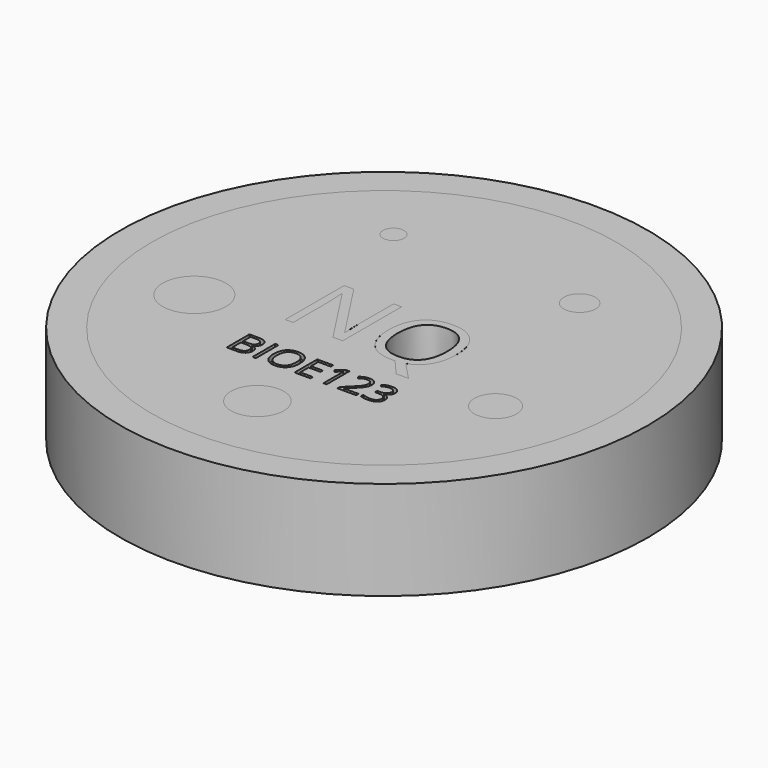
from build123d import *

# Parameters (mm, degrees)
F0_R         = 25
F1_DEPTH     = 3
F2_R         = 25
F2_R_2       = 22
F2_TEXT_SIZE = 9.7620500305
F3_DEPTH     = 6.35
F4_DEPTH     = 6.35
F5_TEXT_SIZE = 3.7660350712
F6_DEPTH     = 0.5


# Not quite as in the source:
# - Text() gives the source's letters only with a copy of the font that has no kerning and outlines rounded to 1/6400 em; it was checked with that copy


with BuildPart() as f1:
    # F0 (on Top) → F1 (new body)
    with BuildSketch(Plane.XY):
        Circle(F0_R)
    extrude(amount=F1_DEPTH)

    # F2 (on face) → F3 (join)
    with BuildSketch(Plane.XY.offset(3)):
        Circle(F2_R)
        Circle(F2_R_2, mode=Mode.SUBTRACT)
        with BuildLine():
            ThreePointArc((-9.6057533582, 11.5208290683), (-8.8167787844, 12.1352549156), (-7.9886185271, 12.6957462967))
            ThreePointArc((-7.9886185271, 12.6957462967), (-9.4045640367, 12.94427191), (-9.6057533582, 11.5208290683))
        make_face()
        with BuildLine():
            ThreePointArc((-9.6057533582, 11.5208290683), (-8.4919515794, 11.1894815353), (-7.8167787844, 12.1352549156))
            ThreePointArc((-7.8167787844, 12.1352549156), (-7.8607034063, 12.4283758315), (-7.9886185271, 12.6957462967))
            ThreePointArc((-7.9886185271, 12.6957462967), (-8.8167787844, 12.1352549156), (-9.6057533582, 11.5208290683))
        make_face()
        with BuildLine():
            ThreePointArc((9.9847025259, 11.1940035496), (8.8167787844, 12.1352549156), (7.560687255, 12.9551537325))
            ThreePointArc((7.560687255, 12.9551537325), (7.9351009059, 10.9217294241), (9.9847025259, 11.1940035496))
        make_face()
        with BuildLine():
            ThreePointArc((10.3167787844, 12.1352549156), (9.2444835342, 13.5729852961), (7.560687255, 12.9551537325))
            ThreePointArc((7.560687255, 12.9551537325), (8.8167787844, 12.1352549156), (9.9847025259, 11.1940035496))
            ThreePointArc((9.9847025259, 11.1940035496), (10.2313256398, 11.6361986123), (10.3167787844, 12.1352549156))
        make_face()
        with BuildLine():
            ThreePointArc((13.5223811584, -6.4919340574), (14.2658477444, -4.6352549156), (14.7556992594, -2.696171242))
            ThreePointArc((14.7556992594, -2.696171242), (12.3637347118, -4.0172209269), (13.5223811584, -6.4919340574))
        make_face()
        with BuildLine():
            ThreePointArc((16.2658477444, -4.6352549156), (15.8437740782, -3.4063739267), (14.7556992594, -2.696171242))
            ThreePointArc((14.7556992594, -2.696171242), (14.2658477444, -4.6352549156), (13.5223811584, -6.4919340574))
            ThreePointArc((13.5223811584, -6.4919340574), (15.3867997568, -6.2915962409), (16.2658477444, -4.6352549156))
        make_face()
        with BuildLine():
            ThreePointArc((2.4913043215, -14.7916666667), (0, -12.5), (-2.4913043215, -14.7916666667))
            ThreePointArc((-2.4913043215, -14.7916666667), (0, -15), (2.4913043215, -14.7916666667))
        make_face()
        with BuildLine():
            ThreePointArc((2.4913043215, -14.7916666667), (0, -15), (-2.4913043215, -14.7916666667))
            ThreePointArc((-2.4913043215, -14.7916666667), (-0.104257365, -17.4978251344), (2.5, -15))
            ThreePointArc((2.5, -15), (2.4978251344, -14.895742635), (2.4913043215, -14.7916666667))
        make_face()
        with BuildLine():
            ThreePointArc((-13.0581267078, -7.3814176744), (-14.2658477444, -4.6352549156), (-14.9029348713, -1.7036819602))
            ThreePointArc((-14.9029348713, -1.7036819602), (-17.1190172933, -5.5623058987), (-13.0581267078, -7.3814176744))
        make_face()
        with BuildLine():
            ThreePointArc((-11.2658477444, -4.6352549156), (-12.3831981993, -2.2995257596), (-14.9029348713, -1.7036819602))
            ThreePointArc((-14.9029348713, -1.7036819602), (-14.2658477444, -4.6352549156), (-13.0581267078, -7.3814176744))
            ThreePointArc((-13.0581267078, -7.3814176744), (-11.7535616232, -6.2748946459), (-11.2658477444, -4.6352549156))
        make_face()
        with Locations((-7.5, -3.5248006052)):
            Text('NQ', F2_TEXT_SIZE, font='Open Sans', text_align=(TextAlign.LEFT, TextAlign.BOTTOM))
    extrude(amount=F3_DEPTH)


with BuildPart() as f4:
    # F2 (on face) → F4 (new body)
    with BuildSketch(Plane.XY.offset(3)):
        Circle(F2_R_2)
        with BuildLine():
            ThreePointArc((-9.6057533582, 11.5208290683), (-9.4045640367, 12.94427191), (-7.9886185271, 12.6957462967))
            ThreePointArc((-7.9886185271, 12.6957462967), (-0.2502086086, 14.9979130432), (7.560687255, 12.9551537325))
            ThreePointArc((7.560687255, 12.9551537325), (9.2444835342, 13.5729852961), (10.3167787844, 12.1352549156))
            ThreePointArc((10.3167787844, 12.1352549156), (10.2313256398, 11.6361986123), (9.9847025259, 11.1940035496))
            ThreePointArc((9.9847025259, 11.1940035496), (13.6888739107, 6.1330849542), (15, 0))
            ThreePointArc((15, 0), (14.9387999667, -1.3536083461), (14.7556992594, -2.696171242))
            ThreePointArc((14.7556992594, -2.696171242), (15.8437740782, -3.4063739267), (16.2658477444, -4.6352549156))
            ThreePointArc((16.2658477444, -4.6352549156), (15.3867997568, -6.2915962409), (13.5223811584, -6.4919340574))
            ThreePointArc((13.5223811584, -6.4919340574), (9.0183657615, -11.9862036939), (2.4913043215, -14.7916666667))
            ThreePointArc((2.4913043215, -14.7916666667), (2.4978251344, -14.895742635), (2.5, -15))
            ThreePointArc((2.5, -15), (-0.104257365, -17.4978251344), (-2.4913043215, -14.7916666667))
            ThreePointArc((-2.4913043215, -14.7916666667), (-8.6124415159, -12.2811176664), (-13.0581267078, -7.3814176744))
            ThreePointArc((-13.0581267078, -7.3814176744), (-17.1190172933, -5.5623058987), (-14.9029348713, -1.7036819602))
            ThreePointArc((-14.9029348713, -1.7036819602), (-13.9244702832, 5.5775556771), (-9.6057533582, 11.5208290683))
        make_face(mode=Mode.SUBTRACT)
        with BuildLine():
            ThreePointArc((-7.9886185271, 12.6957462967), (-7.8607034063, 12.4283758315), (-7.8167787844, 12.1352549156))
            ThreePointArc((-7.8167787844, 12.1352549156), (-8.4919515794, 11.1894815353), (-9.6057533582, 11.5208290683))
            ThreePointArc((-9.6057533582, 11.5208290683), (-13.9244702832, 5.5775556771), (-14.9029348713, -1.7036819602))
            ThreePointArc((-14.9029348713, -1.7036819602), (-12.3831981993, -2.2995257596), (-11.2658477444, -4.6352549156))
            ThreePointArc((-11.2658477444, -4.6352549156), (-11.7535616232, -6.2748946459), (-13.0581267078, -7.3814176744))
            ThreePointArc((-13.0581267078, -7.3814176744), (-8.6124415159, -12.2811176664), (-2.4913043215, -14.7916666667))
            ThreePointArc((-2.4913043215, -14.7916666667), (0, -12.5), (2.4913043215, -14.7916666667))
            ThreePointArc((2.4913043215, -14.7916666667), (9.0183657615, -11.9862036939), (13.5223811584, -6.4919340574))
            ThreePointArc((13.5223811584, -6.4919340574), (12.3637347118, -4.0172209269), (14.7556992594, -2.696171242))
            ThreePointArc((14.7556992594, -2.696171242), (14.9387999667, -1.3536083461), (15, 0))
            ThreePointArc((15, 0), (13.6888739107, 6.1330849542), (9.9847025259, 11.1940035496))
            ThreePointArc((9.9847025259, 11.1940035496), (7.9351009059, 10.9217294241), (7.560687255, 12.9551537325))
            ThreePointArc((7.560687255, 12.9551537325), (-0.2502086086, 14.9979130432), (-7.9886185271, 12.6957462967))
        make_face()
        with BuildLine():
            Line((-1.0982306284, 3.4443879244), (-1.0982306284, -3.5248006052))
            Line((-1.0982306284, -3.5248006052), (-2.0225747407, -3.5248006052))
            Line((-2.0225747407, -3.5248006052), (-5.8312995729, 2.3232774912))
            Line((-5.8312995729, 2.3232774912), (-5.8694325808, 2.3232774912))
            add(Edge.make_bspline(
                [(-5.8694325808, 2.3232774912), (-5.793166565, 1.293686277), (-5.793166565, 0.4364562587)],
                knots=[0, 0, 0, 1, 1, 1], degree=2))
            Line((-5.793166565, 0.4364562587), (-5.793166565, -3.5248006052))
            Line((-5.793166565, -3.5248006052), (-6.5420988408, -3.5248006052))
            Line((-6.5420988408, -3.5248006052), (-6.5420988408, 3.4443879244))
            Line((-6.5420988408, 3.4443879244), (-5.6269066504, 3.4443879244))
            Line((-5.6269066504, 3.4443879244), (-1.8273337401, -2.3808103673))
            Line((-1.8273337401, -2.3808103673), (-1.7892007322, -2.3808103673))
            add(Edge.make_bspline(
                [(-1.7892007322, -2.3808103673), (-1.7983526541, -2.2526834606), (-1.831909701, -1.5540867553)],
                knots=[0, 0, 0, 1, 1, 1], degree=2))
            add(Edge.make_bspline(
                [(-1.831909701, -1.5540867553), (-1.865466748, -0.85549005), (-1.8563148261, -0.5550019475)],
                knots=[0, 0, 0, 1, 1, 1], degree=2))
            Line((-1.8563148261, -0.5550019475), (-1.8563148261, 3.4443879244))
            Line((-1.8563148261, 3.4443879244), (-1.0982306284, 3.4443879244))
        make_face(mode=Mode.SUBTRACT)
        with BuildLine():
            add(Edge.make_bspline(
                [(6.0234899329, 2.6008857889), (6.8669920683, 1.6475605907), (6.8669920683, -0.0302917583)],
                knots=[0, 0, 0, 1, 1, 1], degree=2))
            add(Edge.make_bspline(
                [(6.8669920683, -0.0302917583), (6.8669920683, -1.3695229969), (6.3285539963, -2.2564967614)],
                knots=[0, 0, 0, 1, 1, 1], degree=2))
            add(Edge.make_bspline(
                [(6.3285539963, -2.2564967614), (5.7901159243, -3.1434705259), (4.80780964, -3.4576865112)],
                knots=[0, 0, 0, 1, 1, 1], degree=2))
            Line((4.80780964, -3.4576865112), (6.4658328249, -5.1843491104))
            Line((6.4658328249, -5.1843491104), (5.28828554, -5.1843491104))
            Line((5.28828554, -5.1843491104), (3.9307504576, -3.610218543))
            Line((3.9307504576, -3.610218543), (3.668395363, -3.6208957852))
            add(Edge.make_bspline(
                [(3.668395363, -3.6208957852), (2.1293471629, -3.6208957852), (1.2927089689, -2.6790104893)],
                knots=[0, 0, 0, 1, 1, 1], degree=2))
            add(Edge.make_bspline(
                [(1.2927089689, -2.6790104893), (0.4560707749, -1.7371251934), (0.4560707749, -0.0211398364)],
                knots=[0, 0, 0, 1, 1, 1], degree=2))
            add(Edge.make_bspline(
                [(0.4560707749, -0.0211398364), (0.4560707749, 1.6811176376), (1.2949969494, 2.6176643124)],
                knots=[0, 0, 0, 1, 1, 1], degree=2))
            add(Edge.make_bspline(
                [(1.2949969494, 2.6176643124), (2.1339231239, 3.5542109872), (3.6775472849, 3.5542109872)],
                knots=[0, 0, 0, 1, 1, 1], degree=2))
            add(Edge.make_bspline(
                [(3.6775472849, 3.5542109872), (5.1799877974, 3.5542109872), (6.0234899329, 2.6008857889)],
                knots=[0, 0, 0, 1, 1, 1], degree=2))
        make_face(mode=Mode.SUBTRACT)
    extrude(amount=F4_DEPTH)

    # F5 (on face) → F6 (cut)
    with BuildSketch(Plane.XY.offset(9.35)):
        with Locations((-7.5, -9.7115452513)):
            Text('BIOE123', F5_TEXT_SIZE, font='Open Sans', text_align=(TextAlign.LEFT, TextAlign.BOTTOM))
    extrude(amount=-F6_DEPTH, mode=Mode.SUBTRACT)


solid = Compound([f1.part, f4.part])
